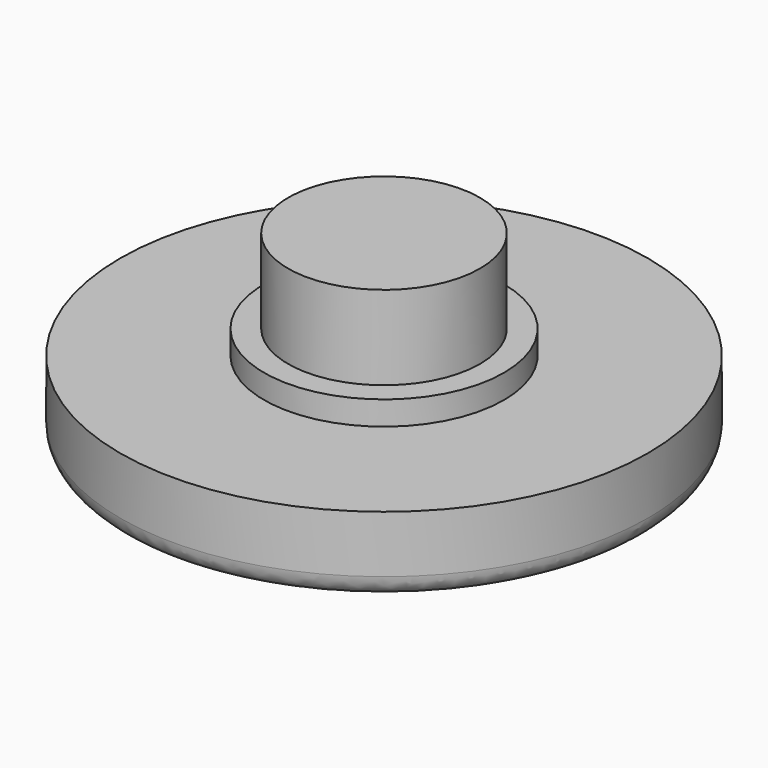
from build123d import *

# Parameters (mm, degrees)
F0_R     = 11
F1_DEPTH = 3.5
F2_R     = 5
F3_DEPTH = 1
F4_R     = 4
F5_DEPTH = 3.5
F6_R     = 1.3518679975
F7_DEPTH = 32.3
F11_R    = 0.9092071391


# Not quite as in the source:
# - a fillet or chamfer that OpenCascade refuses, or shapes differently, is made with other operations: its cross-section is extruded or revolved along the edge and cut away or added
# - a feature names something its author has since deleted; it is built from what else it names


with BuildPart() as f1:
    # F0 (on Top) → F1 (new body)
    with BuildSketch(Plane.XY):
        with Locations((59.4149753451, 64.0600547194)):
            Circle(F0_R)
    extrude(amount=F1_DEPTH)

    # F2 (on face) → F3 (join)
    with BuildSketch(Plane.XY.offset(3.5)):
        with Locations((59.4149753451, 64.0600547194)):
            Circle(F2_R)
    extrude(amount=F3_DEPTH)

    # F4 (on face) → F5 (join)
    with BuildSketch(Plane.XY.offset(4.5)):
        with Locations((59.4149753451, 64.0600547194)):
            Circle(F4_R)
    extrude(amount=F5_DEPTH)

    # F6 (on face) → F7 (join)
    with BuildSketch(Plane(origin=(0, 0, 0), x_dir=(1, 0, 0), z_dir=(0, 0, -1))):
        with Locations((59.4149753451, -64.0600547194)):
            Circle(F6_R)
    extrude(amount=F7_DEPTH)

    # F8 (on face) → F9 (revolve, cut)
    with BuildSketch(Plane(origin=(0, 0, -32.3), x_dir=(1, 0, 0), z_dir=(0, 0, -1))):
        with BuildLine():
            Line((60.7668433426, -64.0600547194), (93.4149753451, -64.0600547194))
            ThreePointArc((93.4149753451, -64.0600547194), (59.4149753451, -30.0600547194), (25.4149753451, -64.0600547194))
            Line((25.4149753451, -64.0600547194), (58.0631073476, -64.0600547194))
            ThreePointArc((58.0631073476, -64.0600547194), (59.4149753451, -62.7081867219), (60.7668433426, -64.0600547194))
        make_face()
        with BuildLine():
            Line((59.4149753451, -64.0600547194), (60.7668433426, -64.0600547194))
            ThreePointArc((60.7668433426, -64.0600547194), (59.4149753451, -62.7081867219), (58.0631073476, -64.0600547194))
            Line((58.0631073476, -64.0600547194), (59.4149753451, -64.0600547194))
        make_face()
    revolve(axis=Axis((76.4149753451, 64.0600547194, -32.3), (1, 0, 0)), mode=Mode.SUBTRACT)

    # F10: fillet of radius 5 on 1 edges, made by hand

    # F10_s1 → F10_t2 (revolve, cut)
    with BuildSketch(Plane.YZ.offset(59.4149753451)):
        with BuildLine():
            ThreePointArc((52.67102491, 0), (53.4091792265, 0.0547873448), (54.1311569369, 0.2179487179))
            ThreePointArc((54.1311569369, 0.2179487179), (53.7867795374, 0.1107978463), (53.4435581222, 0))
            Line((53.4435581222, 0), (52.67102491, 0))
        make_face()
    revolve(axis=Axis((59.4149753451, 64.0600547194, 0), (0, 0, 1)), mode=Mode.SUBTRACT)

    # F11
    f11_edges = [f1.edges().sort_by_distance(p)[0] for p in [
        (51.636801, 71.838229, 0.015157),
        (67.19315, 56.28188, 0.015157),
    ]]
    fillet(f11_edges, radius=F11_R)


solid = f1.part
